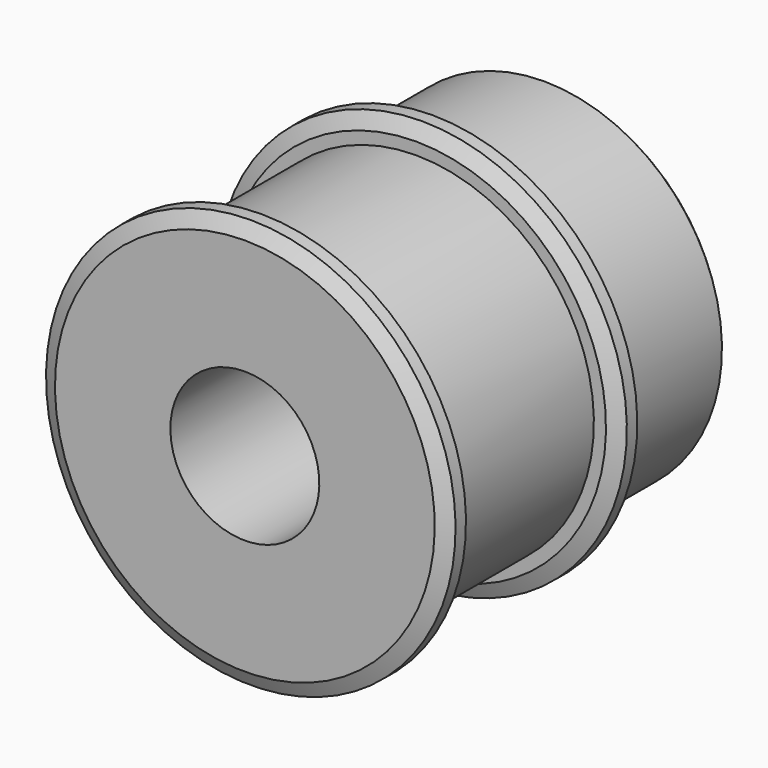
from build123d import *

# Parameters (mm, degrees)
F2_C1_SIZE2 = 0.4
F2_C1_SIZE  = 0.8
F2_C2_SIZE2 = 0.8
F2_C2_SIZE  = 0.4
F2_C3_SIZE2 = 0.8
F2_C3_SIZE  = 0.4
F3_SIZE2    = 0.4
F3_SIZE     = 0.8
F4_SIZE     = 0.4


with BuildPart() as f1:
    # F0 (on Right) → F1 (revolve)
    with BuildSketch(Plane.YZ):
        Polygon((-10.25, 11), (-10.25, 4), (10.25, 4), (10.25, 9.55), (3.25, 9.55), (3.25, 6.35), (2.75, 6.35), (2.75, 11), (1.25, 11), (1.25, 9.55), (-8.75, 9.55), (-8.75, 11), align=None)
    revolve(axis=Axis((0, -3.1587743408, 0), (0, -1, 0)))

    # F2: chamfer of 0.4 x 0.8 on 3 edges, made by hand

    # F2_c1
    f2_c1_edges = [f1.edges().sort_by_distance(p)[0] for p in [
        (0, -10.25, -11),
    ]]
    f2_c1_side = f1.faces().sort_by_distance((0, -10.25, -10.992))[0]
    chamfer(f2_c1_edges, length=F2_C1_SIZE, length2=F2_C1_SIZE2, reference=f2_c1_side)

    # F2_c2
    f2_c2_edges = [f1.edges().sort_by_distance(p)[0] for p in [
        (0, 2.75, -11),
    ]]
    f2_c2_side = f1.faces().sort_by_distance((0, 2.742, -11))[0]
    chamfer(f2_c2_edges, length=F2_C2_SIZE, length2=F2_C2_SIZE2, reference=f2_c2_side)

    # F2_c3
    f2_c3_edges = [f1.edges().sort_by_distance(p)[0] for p in [
        (0, 1.25, -11),
    ]]
    f2_c3_side = f1.faces().sort_by_distance((0, 1.258, -11))[0]
    chamfer(f2_c3_edges, length=F2_C3_SIZE, length2=F2_C3_SIZE2, reference=f2_c3_side)

    # F3
    f3_edges = [f1.edges().sort_by_distance(p)[0] for p in [
        (0, -8.75, -11),
    ]]
    chamfer(f3_edges, length=F3_SIZE, length2=F3_SIZE2)

    # F4
    f4_edges = [f1.edges().sort_by_distance(p)[0] for p in [
        (0, 3.25, -9.55),
        (0, 10.25, -9.55),
    ]]
    chamfer(f4_edges, length=F4_SIZE)


solid = f1.part
